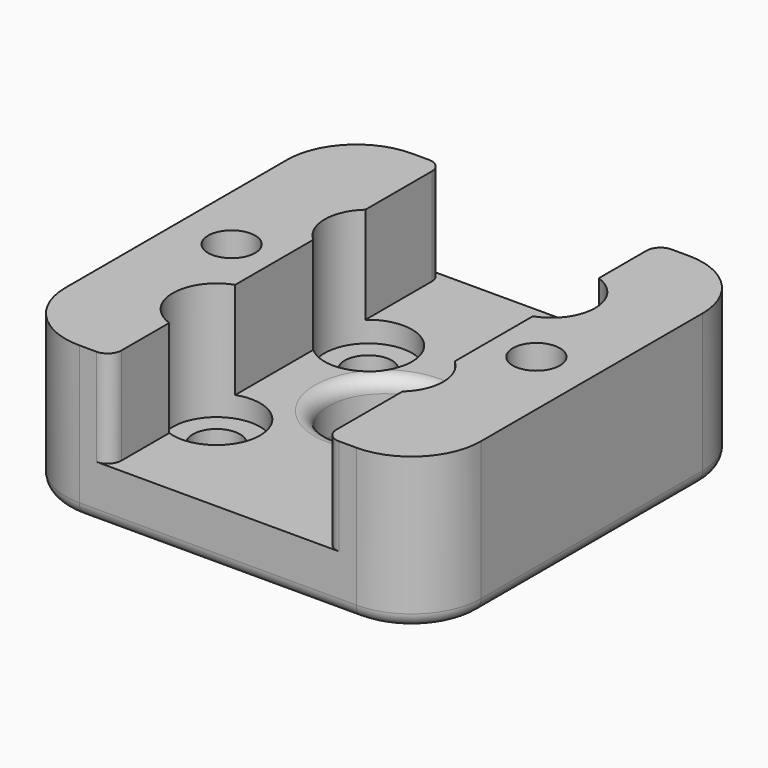
from build123d import *

# Parameters (mm, degrees)
F0_W           = 30
F0_H           = 30
F0_R           = 4
F1_DEPTH       = 11
F3_D           = 3.4
F3_CBORE_D     = 6.3
F3_CBORE_DEPTH = 8.5
F5_D           = 3.4
F6_DEPTH       = 5
F7_R           = 4
F8_DEPTH       = 7
F9_R           = 5
F10_T1_DEPTH   = 9.5
F10_T3_DEPTH   = 20
F10_T5_DEPTH   = 20
F10_T12_ANGLE  = 90
F10_T14_ANGLE  = 90
F10_T16_ANGLE  = 90
F10_T18_ANGLE  = 90


# Not quite as in the source:
# - a fillet or chamfer that OpenCascade refuses, or shapes differently, is made with other operations: its cross-section is extruded or revolved along the edge and cut away or added


with BuildPart() as f1:
    # F0 (on Top) → F1 (new body)
    with BuildSketch(Plane.XY):
        Rectangle(F0_W, F0_H)
        Circle(F0_R, mode=Mode.SUBTRACT)
    extrude(amount=F1_DEPTH)

    # F3 (through all)
    with Locations(Plane.XY.offset(11)):
        with Locations((-6.7175144213, -6.7175144213), (-5.6568542495, 5.6568542495), (6.7175144213, 6.7175144213), (5.6568542495, -5.6568542495)):
            CounterBoreHole(F3_D / 2, F3_CBORE_D / 2, F3_CBORE_DEPTH)

    # F5 (through all)
    with Locations(Plane(origin=(0, 0, 0), x_dir=(1, 0, 0), z_dir=(0, 0, -1))):
        with Locations((-11, 0), (11, 0)):
            Hole(F5_D / 2)

    # F4 (on face) → F6 (cut)
    with BuildSketch(Plane(origin=(0, 0, 0), x_dir=(1, 0, 0), z_dir=(0, 0, -1))):
        Polygon((14, -1.7320508076), (14, 1.7320508076), (11, 3.4641016151), (8, 1.7320508076), (8, -1.7320508076), (11, -3.4641016151), align=None)
        Polygon((-8, -1.7320508076), (-8, 1.7320508076), (-11, 3.4641016151), (-14, 1.7320508076), (-14, -1.7320508076), (-11, -3.4641016151), align=None)
    extrude(amount=-F6_DEPTH, mode=Mode.SUBTRACT)

    # F7 (on face) → F8 (cut)
    with BuildSketch(Plane.XY.offset(11)):
        with BuildLine():
            Line((-7.75, -15), (7.75, -15))
            Line((7.75, -15), (7.75, -8.0108382909))
            ThreePointArc((7.75, -8.0108382909), (2.5068542495, -5.6568542495), (7.75, -3.3028702081))
            Line((7.75, -3.3028702081), (7.75, 3.7415316374))
            ThreePointArc((7.75, 3.7415316374), (3.5675144213, 6.7175144213), (7.75, 9.6934972051))
            Line((7.75, 9.6934972051), (7.75, 15))
            Line((7.75, 15), (-7.75, 15))
            Line((-7.75, 15), (-7.75, 8.0108382909))
            ThreePointArc((-7.75, 8.0108382909), (-4.3666816087, 8.5305199498), (-2.5068542495, 5.6568542495))
            ThreePointArc((-2.5068542495, 5.6568542495), (-4.3666816087, 2.7831885492), (-7.75, 3.3028702081))
            Line((-7.75, 3.3028702081), (-7.75, -3.7415316374))
            ThreePointArc((-7.75, -3.7415316374), (-4.8912928538, -4.1509184682), (-3.5675144213, -6.7175144213))
            ThreePointArc((-3.5675144213, -6.7175144213), (-4.8912928538, -9.2841103744), (-7.75, -9.6934972051))
            Line((-7.75, -9.6934972051), (-7.75, -15))
        make_face()
        Circle(F7_R, mode=Mode.SUBTRACT)
    extrude(amount=-F8_DEPTH, mode=Mode.SUBTRACT)

    # F9
    f9_edges = [f1.edges().sort_by_distance(p)[0] for p in [
        (15, 15, 5.5),
        (-15, 15, 5.5),
        (15, -15, 5.5),
        (-15, -15, 5.5),
    ]]
    fillet(f9_edges, radius=F9_R)

    # F10: fillet of radius 1 on 15 edges, made by hand

    # F10_s2 → F10_t1 (cut)
    with BuildSketch(Plane.XY.offset(4)):
        with BuildLine():
            ThreePointArc((8.75, 15), (8.0428932188, 14.7071067812), (7.75, 14))
            Line((7.75, 14), (7.75, 15))
            Line((7.75, 15), (8.75, 15))
        make_face()
        with BuildLine():
            ThreePointArc((-8.75, 15), (-8.0428932188, 14.7071067812), (-7.75, 14))
            Line((-7.75, 14), (-7.75, 15))
            Line((-7.75, 15), (-8.75, 15))
        make_face()
        with BuildLine():
            ThreePointArc((8.75, -15), (8.0428932188, -14.7071067812), (7.75, -14))
            Line((7.75, -14), (7.75, -15))
            Line((7.75, -15), (8.75, -15))
        make_face()
        with BuildLine():
            ThreePointArc((-8.75, -15), (-8.0428932188, -14.7071067812), (-7.75, -14))
            Line((-7.75, -14), (-7.75, -15))
            Line((-7.75, -15), (-8.75, -15))
        make_face()
    extrude(amount=F10_T1_DEPTH, mode=Mode.SUBTRACT)

    # F10_s4 → F10_t3 (cut)
    with BuildSketch(Plane.YZ.offset(-10)):
        with BuildLine():
            ThreePointArc((-15, 1), (-14.7071067812, 0.2928932188), (-14, 0))
            Line((-14, 0), (-15, 0))
            Line((-15, 0), (-15, 1))
        make_face()
        with BuildLine():
            ThreePointArc((14, 0), (14.7071067812, 0.2928932188), (15, 1))
            Line((15, 1), (15, 0))
            Line((15, 0), (14, 0))
        make_face()
    extrude(amount=F10_T3_DEPTH, mode=Mode.SUBTRACT)

    # F10_s6 → F10_t5 (cut)
    with BuildSketch(Plane.XZ.offset(-10)):
        with BuildLine():
            ThreePointArc((-14, 0), (-14.7071067812, 0.2928932188), (-15, 1))
            Line((-15, 1), (-15, 0))
            Line((-15, 0), (-14, 0))
        make_face()
        with BuildLine():
            ThreePointArc((14, 0), (14.7071067812, 0.2928932188), (15, 1))
            Line((15, 1), (15, 0))
            Line((15, 0), (14, 0))
        make_face()
    extrude(amount=F10_T5_DEPTH, mode=Mode.SUBTRACT)

    # F10_s7 → F10_t8 (revolve, cut)
    with BuildSketch(Plane.XZ):
        with BuildLine():
            ThreePointArc((5, 4), (4.2928932188, 3.7071067812), (4, 3))
            Line((4, 3), (4, 4))
            Line((4, 4), (5, 4))
        make_face()
    revolve(axis=Axis((0, 0, 4), (0, 0, 1)), mode=Mode.SUBTRACT)

    # F10_s9 → F10_t10 (revolve, cut)
    with BuildSketch(Plane.XZ):
        with BuildLine():
            ThreePointArc((5, 0), (4.2928932188, 0.2928932188), (4, 1))
            Line((4, 1), (4, 0))
            Line((4, 0), (5, 0))
        make_face()
    revolve(axis=Axis((0, 0, 0), (0, 0, 1)), mode=Mode.SUBTRACT)

    # F10_s11 → F10_t12 (revolve, cut)
    with BuildSketch(Plane.YZ.offset(-10)):
        with BuildLine():
            ThreePointArc((-14, 0), (-14.7071067812, 0.2928932188), (-15, 1))
            Line((-15, 1), (-15, 0))
            Line((-15, 0), (-14, 0))
        make_face()
    revolve(axis=Axis((-10, -10, 0), (0, 0, -1)), revolution_arc=F10_T12_ANGLE, mode=Mode.SUBTRACT)

    # F10_s13 → F10_t14 (revolve, cut)
    with BuildSketch(Plane.YZ.offset(10)):
        with BuildLine():
            ThreePointArc((-14, 0), (-14.7071067812, 0.2928932188), (-15, 1))
            Line((-15, 1), (-15, 0))
            Line((-15, 0), (-14, 0))
        make_face()
    revolve(axis=Axis((10, -10, 0), (0, 0, 1)), revolution_arc=F10_T14_ANGLE, mode=Mode.SUBTRACT)

    # F10_s15 → F10_t16 (revolve, cut)
    with BuildSketch(Plane.XZ.offset(-10)):
        with BuildLine():
            ThreePointArc((-14, 0), (-14.7071067812, 0.2928932188), (-15, 1))
            Line((-15, 1), (-15, 0))
            Line((-15, 0), (-14, 0))
        make_face()
    revolve(axis=Axis((-10, 10, 0), (0, 0, -1)), revolution_arc=F10_T16_ANGLE, mode=Mode.SUBTRACT)

    # F10_s17 → F10_t18 (revolve, cut)
    with BuildSketch(Plane.XZ.offset(-10)):
        with BuildLine():
            ThreePointArc((14, 0), (14.7071067812, 0.2928932188), (15, 1))
            Line((15, 1), (15, 0))
            Line((15, 0), (14, 0))
        make_face()
    revolve(axis=Axis((10, 10, 0), (0, 0, 1)), revolution_arc=F10_T18_ANGLE, mode=Mode.SUBTRACT)


solid = f1.part
